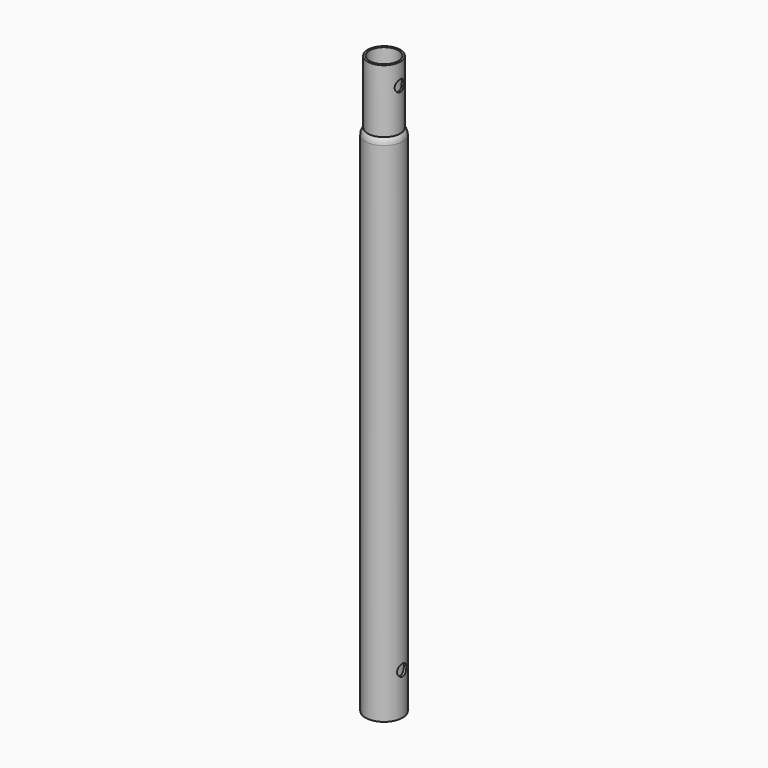
from build123d import *

# Parameters (mm, degrees)
F0_R          = 9.7
F1_DEPTH      = 268
F2_R          = 8.5
F3_DEPTH      = 33
F5_R          = 7.5
F6_DEPTH      = 36.4
F7_R          = 8.5
F8_DEPTH      = 267
F4_R          = 3
F9_DEPTH      = 25
F9_DEPTH_BACK = 25


# Not quite as in the source:
# - a fillet or chamfer that OpenCascade refuses, or shapes differently, is made with other operations: its cross-section is extruded or revolved along the edge and cut away or added


with BuildPart() as f1:
    # F0 (on Top) → F1 (new body)
    with BuildSketch(Plane.XY):
        Circle(F0_R)
    extrude(amount=F1_DEPTH)

    # F2 (on face) → F3 (join)
    with BuildSketch(Plane.XY.offset(268)):
        Circle(F2_R)
    extrude(amount=F3_DEPTH)

    # F5 (on face) → F6 (cut)
    with BuildSketch(Plane.XY.offset(301)):
        Circle(F5_R)
    extrude(amount=-F6_DEPTH, mode=Mode.SUBTRACT)

    # F7 (on face) → F8 (cut)
    with BuildSketch(Plane(origin=(0, 0, 0), x_dir=(1, 0, 0), z_dir=(0, 0, -1))):
        Circle(F7_R)
    extrude(amount=-F8_DEPTH, mode=Mode.SUBTRACT)

    # F4 (on Right) → F9 (cut, two sides)
    with BuildSketch(Plane.YZ) as f9_sk:
        with Locations((0, 22)):
            Circle(F4_R)
        with Locations((0, 290)):
            Circle(F4_R)
    extrude(amount=-F9_DEPTH, mode=Mode.SUBTRACT)
    extrude(f9_sk.sketch, amount=F9_DEPTH_BACK, mode=Mode.SUBTRACT)

    # F10: fillet of radius 5 on 1 edges, made by hand

    # F10_s1 → F10_t2 (revolve, cut)
    with BuildSketch(Plane.XZ):
        with BuildLine():
            add(Edge.make_bspline(
                [(9.7, 264.7503846381), (9.7, 266.5967570028), (8.5, 268)],
                knots=[0, 0, 0, 1, 1, 1], degree=2, weights=[1, 1, 1]))
            Line((8.5, 268), (8.576, 268.0649923072))
            ThreePointArc((8.576, 268.0649923072), (9.1, 268.1), (9.7, 268.1))
            Line((9.7, 268.1), (9.8, 268))
            Line((9.8, 268), (9.8, 264.7503846381))
            Line((9.8, 264.7503846381), (9.7, 264.7503846381))
        make_face()
    revolve(axis=Axis((0, 0, 268), (0, 0, 1)), mode=Mode.SUBTRACT)


solid = f1.part
